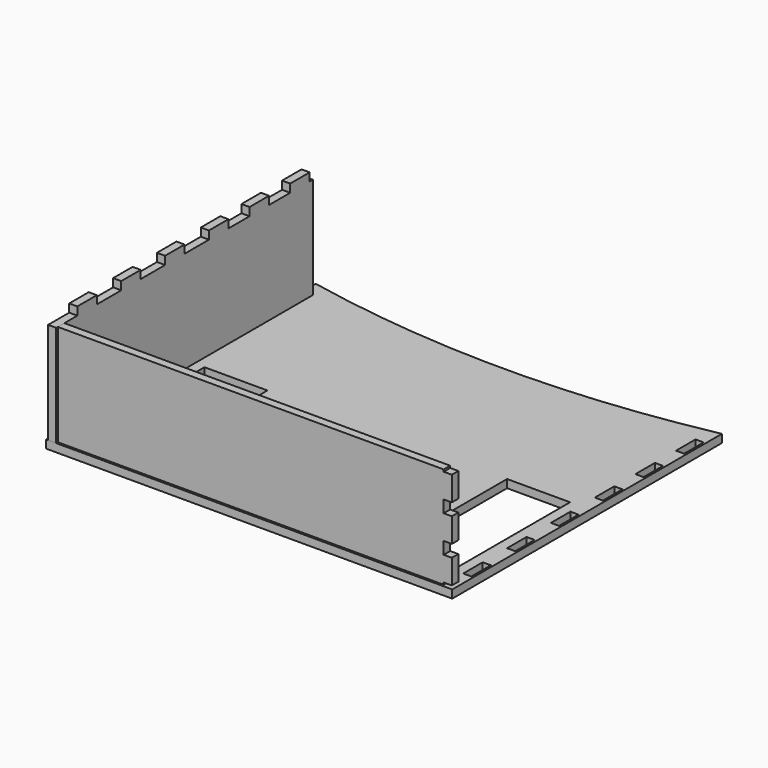
from build123d import *

# Parameters (mm, degrees)
F0_W      = 12
F0_H      = 4
F0_W_2    = 4
F0_H_2    = 12
F1_DEPTH  = 2
F2_W      = 4
F2_H      = 12
F3_DEPTH  = 4
F2_H_2    = 15
F2_H_3    = 13
F4_DEPTH  = 50
F6_W      = 4
F6_H      = 12
F7_DEPTH  = 4
F8_W      = 4
F8_H      = 12
F9_DEPTH  = 4
F10_W     = 12
F10_H     = 4
F11_DEPTH = 4
F10_W_2   = 190
F12_DEPTH = 50
F13_W     = 4
F13_H     = 12
F14_DEPTH = 4
F15_W     = 4
F15_H     = 12
F16_DEPTH = 4
F17_W     = 12
F17_H     = 4
F17_W_2   = 4
F17_H_2   = 12
F18_DEPTH = 4
F19_W     = 31
F19_H     = 75
F20_DEPTH = 4
F22_W     = 4
F22_H     = 13
F22_H_2   = 12
F22_H_3   = 1.9699091613
F23_DEPTH = 50
F24_W     = 4
F24_H     = 12
F25_DEPTH = 4
F26_W     = 4
F26_H     = 12
F27_DEPTH = 4


# Not quite as in the source:
# - a feature names something its author has since deleted; it is built from what else it names


with BuildPart() as f1:
    # F0 (on Top) → F1 (new body, symmetric)
    with BuildSketch(Plane.XY):
        with BuildLine():
            Line((-100, -100), (100, -100))
            Line((100, -100), (100, 66))
            ThreePointArc((100, 66), (0, 55.8979485566), (-100, 66))
            Line((-100, 66), (-100, -100))
        make_face()
        with Locations((-88, -97)):
            Rectangle(F0_W, F0_H, mode=Mode.SUBTRACT)
        with Locations((-97, -81)):
            Rectangle(F0_W_2, F0_H_2, mode=Mode.SUBTRACT)
        with Locations((-63, -97)):
            Rectangle(F0_W, F0_H, mode=Mode.SUBTRACT)
        with Locations((-97, -54)):
            Rectangle(F0_W_2, F0_H_2, mode=Mode.SUBTRACT)
        with Locations((-38, -97)):
            Rectangle(F0_W, F0_H, mode=Mode.SUBTRACT)
        with Locations((-13, -97)):
            Rectangle(F0_W, F0_H, mode=Mode.SUBTRACT)
        with Locations((-97, -27)):
            Rectangle(F0_W_2, F0_H_2, mode=Mode.SUBTRACT)
        with Locations((13, -97)):
            Rectangle(F0_W, F0_H, mode=Mode.SUBTRACT)
        with Locations((38, -97)):
            Rectangle(F0_W, F0_H, mode=Mode.SUBTRACT)
        with Locations((63, -97)):
            Rectangle(F0_W, F0_H, mode=Mode.SUBTRACT)
        with Locations((88, -97)):
            Rectangle(F0_W, F0_H, mode=Mode.SUBTRACT)
        with Locations((97, -81)):
            Rectangle(F0_W_2, F0_H_2, mode=Mode.SUBTRACT)
        with Locations((97, -54)):
            Rectangle(F0_W_2, F0_H_2, mode=Mode.SUBTRACT)
        with Locations((97, -27)):
            Rectangle(F0_W_2, F0_H_2, mode=Mode.SUBTRACT)
        with Locations((-97, 0)):
            Rectangle(F0_W_2, F0_H_2, mode=Mode.SUBTRACT)
        with Locations((-97, 25)):
            Rectangle(F0_W_2, F0_H_2, mode=Mode.SUBTRACT)
        with Locations((-97, 50)):
            Rectangle(F0_W_2, F0_H_2, mode=Mode.SUBTRACT)
        with Locations((97, 0)):
            Rectangle(F0_W_2, F0_H_2, mode=Mode.SUBTRACT)
        with Locations((97, 25)):
            Rectangle(F0_W_2, F0_H_2, mode=Mode.SUBTRACT)
        with Locations((97, 50)):
            Rectangle(F0_W_2, F0_H_2, mode=Mode.SUBTRACT)
    extrude(amount=F1_DEPTH, both=True)


with BuildPart() as f3:
    # F2 (on face) → F3 (new body, through all)
    with BuildSketch(Plane.XY.offset(2)):
        with Locations((-97, 0)):
            Rectangle(F2_W, F2_H)
    extrude(amount=-F3_DEPTH)



with BuildPart() as f3b:
    # F2 (on face) → F3, piece 2 (new body, through all)
    with BuildSketch(Plane.XY.offset(2)):
        with Locations((-97, -27)):
            Rectangle(F2_W, F2_H)
    extrude(amount=-F3_DEPTH)


with BuildPart() as f3c:
    # F2 (on face) → F3, piece 3 (new body, through all)
    with BuildSketch(Plane.XY.offset(2)):
        with Locations((-97, -54)):
            Rectangle(F2_W, F2_H)
    extrude(amount=-F3_DEPTH)


with BuildPart() as f3d:
    # F2 (on face) → F3, piece 4 (new body, through all)
    with BuildSketch(Plane.XY.offset(2)):
        with Locations((-97, -81)):
            Rectangle(F2_W, F2_H)
    extrude(amount=-F3_DEPTH)


with BuildPart() as f3_1:
    add(f3.part)

    add(f3b.part)  # F4 merges F3b

    add(f3c.part)  # F4 merges F3c

    add(f3d.part)  # F4 merges F3d
    # F2 (on face) → F4 (join)
    with BuildSketch(Plane.XY.offset(2)):
        with Locations((-97, 0)):
            Rectangle(F2_W, F2_H)
        with Locations((-97, -13.5)):
            Rectangle(F2_W, F2_H_2)
        with Locations((-97, -27)):
            Rectangle(F2_W, F2_H)
        with Locations((-97, -40.5)):
            Rectangle(F2_W, F2_H_2)
        with Locations((-97, -54)):
            Rectangle(F2_W, F2_H)
        with Locations((-97, -67.5)):
            Rectangle(F2_W, F2_H_2)
        with Locations((-97, -81)):
            Rectangle(F2_W, F2_H)
        with Locations((-97, -93.5)):
            Rectangle(F2_W, F2_H_3)
    extrude(amount=F4_DEPTH)

    # F5: union 

    # F6 (on face) → F7 (join)
    with BuildSketch(Plane.XY.offset(52)):
        with Locations((-97, 0)):
            Rectangle(F6_W, F6_H)
        with Locations((-97, -27)):
            Rectangle(F6_W, F6_H)
        with Locations((-97, -54)):
            Rectangle(F6_W, F6_H)
        with Locations((-97, -81)):
            Rectangle(F6_W, F6_H)
    extrude(amount=F7_DEPTH)

    # F8 (on face) → F9 (cut, through all)
    with BuildSketch(Plane.YZ.offset(-95)):
        with Locations((-97, 45)):
            Rectangle(F8_W, F8_H)
        with Locations((-97, 27)):
            Rectangle(F8_W, F8_H)
        with Locations((-97, 9)):
            Rectangle(F8_W, F8_H)
    extrude(amount=-F9_DEPTH, mode=Mode.SUBTRACT)

    # F22 (on face) → F23 (join)
    with BuildSketch(Plane.XY.offset(2)):
        with Locations((-97, 12.5)):
            Rectangle(F22_W, F22_H)
        with Locations((-97, 0)):
            Rectangle(F22_W, F22_H_2)
        with Locations((-97, 25)):
            Rectangle(F22_W, F22_H_2)
        with Locations((-97, 37.5)):
            Rectangle(F22_W, F22_H)
        with Locations((-97, 50)):
            Rectangle(F22_W, F22_H_2)
        with Locations((-97, 56.9849545807)):
            Rectangle(F22_W, F22_H_3)
    extrude(amount=F23_DEPTH)

    # F24 (on face) → F25 (join)
    with BuildSketch(Plane.XY.offset(52)):
        with Locations((-97, 25)):
            Rectangle(F24_W, F24_H)
        with Locations((-97, 50)):
            Rectangle(F24_W, F24_H)
    extrude(amount=F25_DEPTH)

    # F26 (on face) → F27 (join, through all)
    with BuildSketch(Plane(origin=(0, 0, 2), x_dir=(1, 0, 0), z_dir=(0, 0, -1))):
        with Locations((-97, -50)):
            Rectangle(F26_W, F26_H)
        with Locations((-97, -25)):
            Rectangle(F26_W, F26_H)
    extrude(amount=F27_DEPTH)


with BuildPart() as f11:
    # F10 (on face) → F11 (new body, through all)
    with BuildSketch(Plane.XY.offset(2)):
        with Locations((-88, -97)):
            Rectangle(F10_W, F10_H)
    extrude(amount=-F11_DEPTH)



with BuildPart() as f11b:
    # F10 (on face) → F11, piece 2 (new body, through all)
    with BuildSketch(Plane.XY.offset(2)):
        with Locations((-63, -97)):
            Rectangle(F10_W, F10_H)
    extrude(amount=-F11_DEPTH)


with BuildPart() as f11c:
    # F10 (on face) → F11, piece 3 (new body, through all)
    with BuildSketch(Plane.XY.offset(2)):
        with Locations((-38, -97)):
            Rectangle(F10_W, F10_H)
    extrude(amount=-F11_DEPTH)


with BuildPart() as f11d:
    # F10 (on face) → F11, piece 4 (new body, through all)
    with BuildSketch(Plane.XY.offset(2)):
        with Locations((-13, -97)):
            Rectangle(F10_W, F10_H)
    extrude(amount=-F11_DEPTH)


with BuildPart() as f11e:
    # F10 (on face) → F11, piece 5 (new body, through all)
    with BuildSketch(Plane.XY.offset(2)):
        with Locations((13, -97)):
            Rectangle(F10_W, F10_H)
    extrude(amount=-F11_DEPTH)


with BuildPart() as f11f:
    # F10 (on face) → F11, piece 6 (new body, through all)
    with BuildSketch(Plane.XY.offset(2)):
        with Locations((38, -97)):
            Rectangle(F10_W, F10_H)
    extrude(amount=-F11_DEPTH)


with BuildPart() as f11g:
    # F10 (on face) → F11, piece 7 (new body, through all)
    with BuildSketch(Plane.XY.offset(2)):
        with Locations((63, -97)):
            Rectangle(F10_W, F10_H)
    extrude(amount=-F11_DEPTH)


with BuildPart() as f11h:
    # F10 (on face) → F11, piece 8 (new body, through all)
    with BuildSketch(Plane.XY.offset(2)):
        with Locations((88, -97)):
            Rectangle(F10_W, F10_H)
    extrude(amount=-F11_DEPTH)


with BuildPart() as f11_1:
    add(f11.part)

    add(f11b.part)  # F12 merges F11b

    add(f11c.part)  # F12 merges F11c

    add(f11d.part)  # F12 merges F11d

    add(f11e.part)  # F12 merges F11e

    add(f11f.part)  # F12 merges F11f

    add(f11g.part)  # F12 merges F11g

    add(f11h.part)  # F12 merges F11h
    # F10 (on face) → F12 (join)
    with BuildSketch(Plane.XY.offset(2)):
        with Locations((0, -97)):
            Rectangle(F10_W_2, F10_H)
    extrude(amount=F12_DEPTH)

    # F13 (on face) → F14 (join)
    with BuildSketch(Plane(origin=(-95, 0, 0), x_dir=(0, -1, 0), z_dir=(-1, 0, 0))):
        with Locations((97, 45)):
            Rectangle(F13_W, F13_H)
        with Locations((97, 27)):
            Rectangle(F13_W, F13_H)
        with Locations((97, 9)):
            Rectangle(F13_W, F13_H)
    extrude(amount=F14_DEPTH)

    # F15 (on face) → F16 (join)
    with BuildSketch(Plane.YZ.offset(95)):
        with Locations((-97, 45)):
            Rectangle(F15_W, F15_H)
        with Locations((-97, 27)):
            Rectangle(F15_W, F15_H)
        with Locations((-97, 9)):
            Rectangle(F15_W, F15_H)
    extrude(amount=F16_DEPTH)


with BuildPart() as f18:
    # F17 (on face) → F18 (new body)
    with BuildSketch(Plane.XY.offset(2)):
        with BuildLine():
            Line((-100, -100), (100, -100))
            Line((100, -100), (100, 6))
            ThreePointArc((100, 6), (78.6066430413, 36.5387320014), (48.2820539811, 58.23456507))
            ThreePointArc((48.2820539811, 58.23456507), (0, 55.8979485566), (-48.2820539811, 58.23456507))
            ThreePointArc((-48.2820539811, 58.23456507), (-78.6066430413, 36.5387320014), (-100, 6))
            Line((-100, 6), (-100, -100))
        make_face()
        with Locations((-88, -97)):
            Rectangle(F17_W, F17_H, mode=Mode.SUBTRACT)
        with Locations((-97, -81)):
            Rectangle(F17_W_2, F17_H_2, mode=Mode.SUBTRACT)
        with Locations((-63, -97)):
            Rectangle(F17_W, F17_H, mode=Mode.SUBTRACT)
        with Locations((-97, -54)):
            Rectangle(F17_W_2, F17_H_2, mode=Mode.SUBTRACT)
        with Locations((-38, -97)):
            Rectangle(F17_W, F17_H, mode=Mode.SUBTRACT)
        with Locations((-13, -97)):
            Rectangle(F17_W, F17_H, mode=Mode.SUBTRACT)
        with Locations((-97, -27)):
            Rectangle(F17_W_2, F17_H_2, mode=Mode.SUBTRACT)
        with Locations((13, -97)):
            Rectangle(F17_W, F17_H, mode=Mode.SUBTRACT)
        with Locations((38, -97)):
            Rectangle(F17_W, F17_H, mode=Mode.SUBTRACT)
        with Locations((63, -97)):
            Rectangle(F17_W, F17_H, mode=Mode.SUBTRACT)
        with Locations((88, -97)):
            Rectangle(F17_W, F17_H, mode=Mode.SUBTRACT)
        with Locations((97, -81)):
            Rectangle(F17_W_2, F17_H_2, mode=Mode.SUBTRACT)
        with Locations((97, -54)):
            Rectangle(F17_W_2, F17_H_2, mode=Mode.SUBTRACT)
        with Locations((97, -27)):
            Rectangle(F17_W_2, F17_H_2, mode=Mode.SUBTRACT)
        with Locations((-97, 0)):
            Rectangle(F17_W_2, F17_H_2, mode=Mode.SUBTRACT)
        with Locations((97, 0)):
            Rectangle(F17_W_2, F17_H_2, mode=Mode.SUBTRACT)
    extrude(amount=-F18_DEPTH)


with BuildPart() as f20_tool:
    # F19 (on face) → F20 (new body, through all)
    with BuildSketch(Plane.XY.offset(2)):
        with Locations((-74.5, -52.5)):
            Rectangle(F19_W, F19_H)
        with Locations((74.5, -52.5)):
            Rectangle(F19_W, F19_H)
    extrude(amount=-F20_DEPTH)


with BuildPart() as f1_1:
    add(f1.part)

    # F20: cut by f20_tool
    add(f20_tool.part, mode=Mode.SUBTRACT)


with BuildPart() as f18_1:
    add(f18.part)

    # F20: cut by f20_tool
    add(f20_tool.part, mode=Mode.SUBTRACT)


solid = Compound([f3_1.part, f11_1.part, f1_1.part])
